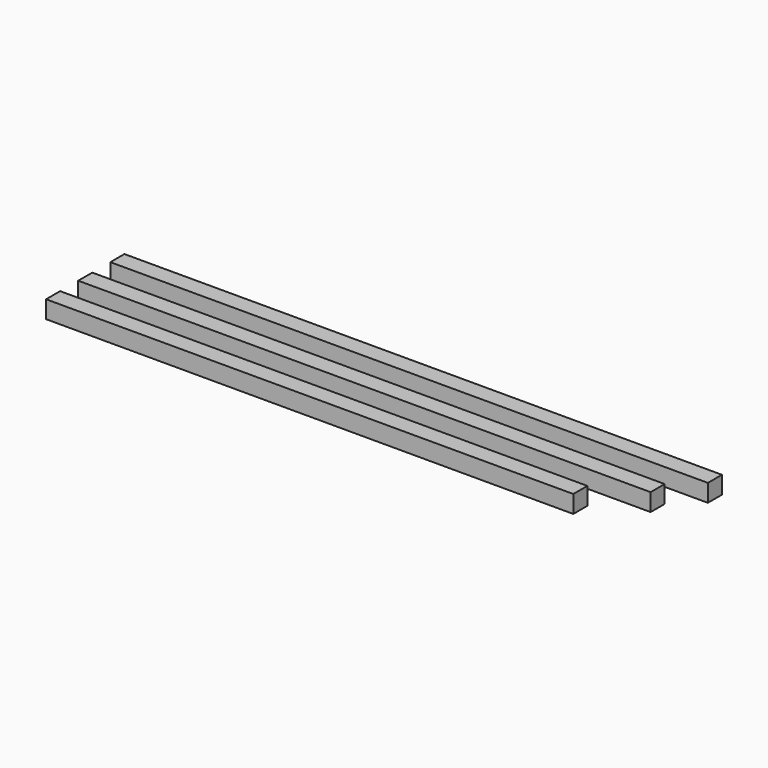
from build123d import *

# Parameters (mm, degrees)
F0_W     = 88.9
F0_H     = 88.9
F1_DEPTH = 2667
F3_DEPTH = 228.6
F5_DEPTH = 355.6


with BuildPart() as f1:
    # F0 (on Right) → F1 (new body)
    with BuildSketch(Plane.YZ):
        Rectangle(F0_W, F0_H)
    extrude(amount=F1_DEPTH)


with BuildPart() as f2_1:
    # F2: copy of F1
    add(f1.part.moved(Location((0, 203.2, 0))))

    # F3 (add): a face of the model
    f3_faces = [f2_1.faces().sort_by_distance(p)[0] for p in [
        (2667, 203.2, 0),
    ]]
    extrude(f3_faces, amount=F3_DEPTH)


with BuildPart() as f4_1:
    # F4: copy of F1
    add(f1.part.moved(Location((0, 406.4, 0))))

    # F5 (add): a face of the model
    f5_faces = [f4_1.faces().sort_by_distance(p)[0] for p in [
        (2667, 406.4, 0),
    ]]
    extrude(f5_faces, amount=F5_DEPTH)


solid = Compound([f1.part, f2_1.part, f4_1.part])
